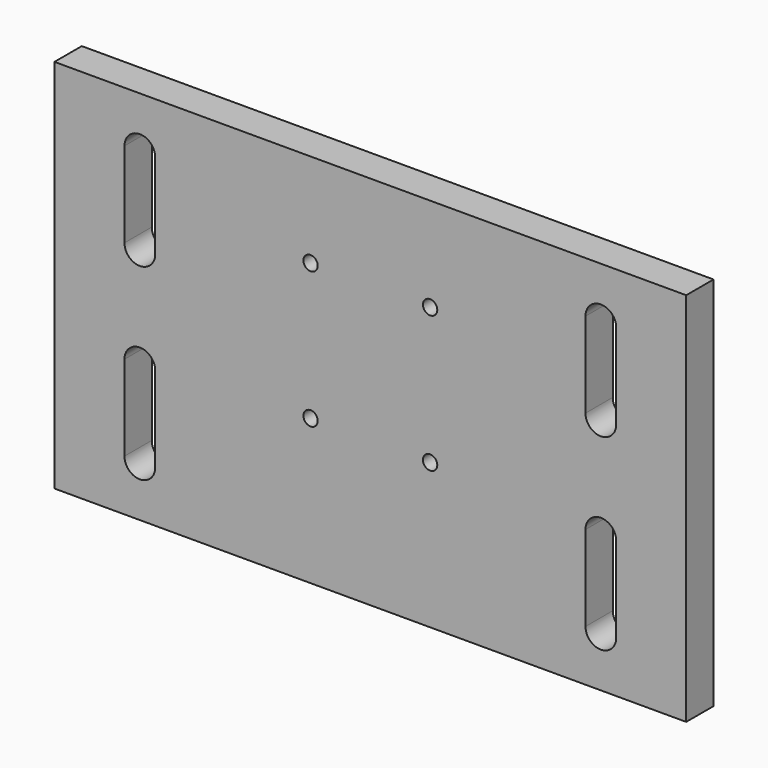
from build123d import *

# Parameters (mm, degrees)
F0_W     = 185
F0_H     = 110
F1_DEPTH = 5
F3_DEPTH = 10.001
F5_D     = 4.2
F5_DEPTH = 17.4
F5_TIP   = 1.2618073


with BuildPart() as f1:
    # F0 (on Front) → F1 (new body, symmetric)
    with BuildSketch(Plane.XZ):
        Rectangle(F0_W, F0_H)
    extrude(amount=F1_DEPTH, both=True)

    # F2 (on face) → F3 (cut, through all)
    with BuildSketch(Plane.XZ.offset(5)):
        with BuildLine():
            ThreePointArc((-63, 40), (-67.5, 44.5), (-72, 40))
            Line((-72, 40), (-72, 15))
            ThreePointArc((-72, 15), (-67.5, 10.5), (-63, 15))
            Line((-63, 15), (-63, 40))
        make_face()
        with BuildLine():
            ThreePointArc((-63, -15), (-67.5, -10.5), (-72, -15))
            Line((-72, -15), (-72, -40))
            ThreePointArc((-72, -40), (-67.5, -44.5), (-63, -40))
            Line((-63, -40), (-63, -15))
        make_face()
        with BuildLine():
            ThreePointArc((72, 40), (67.5, 44.5), (63, 40))
            Line((63, 40), (63, 15))
            ThreePointArc((63, 15), (67.5, 10.5), (72, 15))
            Line((72, 15), (72, 40))
        make_face()
        with BuildLine():
            ThreePointArc((72, -15), (67.5, -10.5), (63, -15))
            Line((63, -15), (63, -40))
            ThreePointArc((63, -40), (67.5, -44.5), (72, -40))
            Line((72, -40), (72, -15))
        make_face()
    extrude(amount=-F3_DEPTH, mode=Mode.SUBTRACT)

    # F5
    with Locations(Plane.XZ.offset(5)):
        with Locations((-17.5, 27.5), (-17.5, -12.5), (17.5, 27.5), (17.5, -12.5)):
            Hole(F5_D / 2, depth=F5_DEPTH)
            with Locations((0, 0, -(F5_DEPTH + F5_TIP / 2))):  # 118° drill point
                Cone(0, F5_D / 2, F5_TIP, mode=Mode.SUBTRACT)


solid = f1.part
